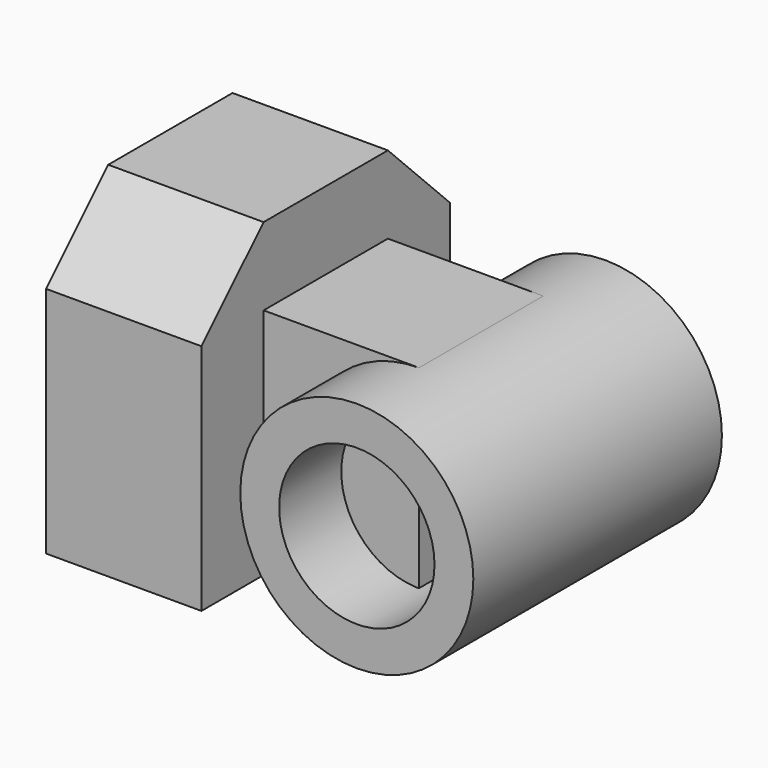
from build123d import *

# Parameters (mm, degrees)
F1_DEPTH = 12.7
F2_W     = 12.7
F2_H     = 19.05
F3_DEPTH = 25.4
F4_R     = 9.525
F5_DEPTH = 25.4
F6_R     = 6.35
F7_DEPTH = 25.4


with BuildPart() as f1:
    # F0 (on Right) → F1 (new body)
    with BuildSketch(Plane.YZ):
        Polygon((0, 19.05), (0, 0), (25.4, 0), (25.4, 19.05), (19.05, 25.4), (6.35, 25.4), align=None)
    extrude(amount=F1_DEPTH)

    # F2 (on Right) → F3 (join)
    with BuildSketch(Plane.YZ):
        with Locations((12.7, 9.525)):
            Rectangle(F2_W, F2_H)
    extrude(amount=F3_DEPTH)


with BuildPart() as f5:
    # F4 (on Front) → F5 (new body)
    with BuildSketch(Plane.XZ):
        with Locations((25.4, 9.525)):
            Circle(F4_R)
    extrude(amount=-F5_DEPTH)

    # F6 (on face) → F7 (cut)
    with BuildSketch(Plane.XZ):
        with Locations((25.4, 9.525)):
            Circle(F6_R)
    extrude(amount=-F7_DEPTH, mode=Mode.SUBTRACT)


solid = Compound([f1.part, f5.part])
